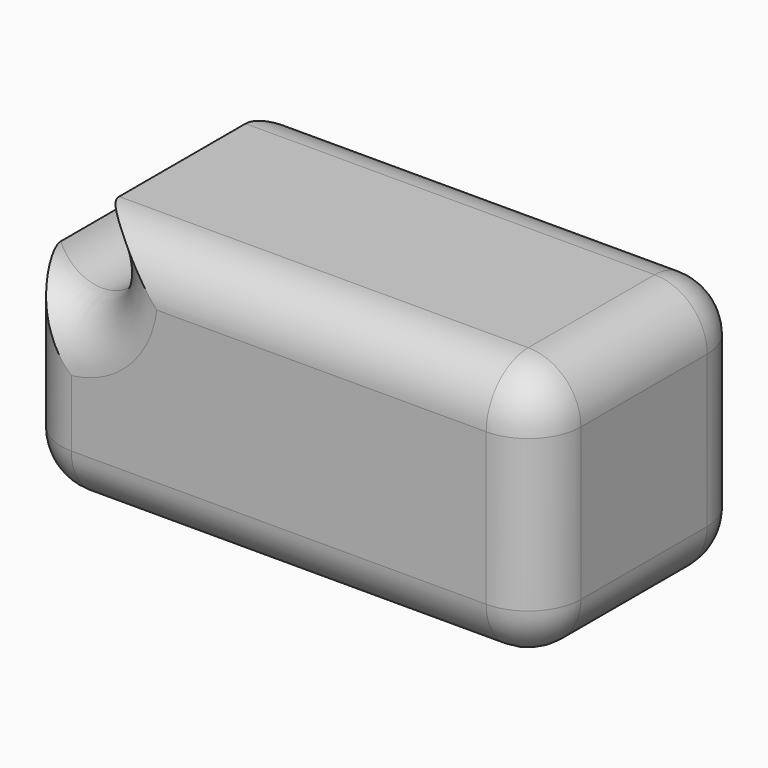
from build123d import *

# Parameters (mm, degrees)
F1_DEPTH     = 25.4
F2_T1_DEPTH  = 69.9704050186
F2_T3_DEPTH  = 26.8039856385
F2_T5_DEPTH  = 57.8223550216
F2_T7_DEPTH  = 50.2159356415
F2_T9_DEPTH  = 15.24
F2_S13_W     = 5.08
F2_S13_H     = 5.08
F2_T14_DEPTH = 5.08
F2_S19_W     = 5.08
F2_S19_H     = 5.08
F2_T20_DEPTH = 5.08
F2_T24_ANGLE = 359.64
F3_T1_DEPTH  = 15.24
F3_T3_DEPTH  = 52.1904050186
F3_S7_W      = 5.08
F3_S7_H      = 5.08
F3_T8_DEPTH  = 5.08
F3_T12_ANGLE = 89.9999999979
F4_T1_DEPTH  = 15.24
F4_S5_W      = 5.08
F4_S5_H      = 5.08
F4_T6_DEPTH  = 5.08
F4_S11_W     = 5.08
F4_S11_H     = 5.08
F4_T12_DEPTH = 5.08


# Not quite as in the source:
# - a fillet or chamfer that OpenCascade refuses, or shapes differently, is made with other operations: its cross-section is extruded or revolved along the edge and cut away or added


with BuildPart() as f1:
    # F0 (on Front) → F1 (new body)
    with BuildSketch(Plane.XZ):
        with BuildLine():
            Line((3.1376483385, 38.9353483915), (-41.4327566801, 38.9353483915))
            ThreePointArc((-41.4327566801, 38.9353483915), (-39.4863101259, 37.3460437845), (-38.7548631728, 34.9419787526))
            ThreePointArc((-38.7548631728, 34.9419787526), (-42.236270886, 30.7070512215), (-47.0647066832, 33.3033983885))
            Line((-47.0647066832, 33.3033983885), (-47.0647066832, 14.11941275))
            Line((-47.0647066832, 14.11941275), (3.1376483385, 14.11941275))
            Line((3.1376483385, 14.11941275), (3.1376483385, 38.9353483915))
        make_face()
    extrude(amount=F1_DEPTH)

    # F2: fillet of radius 5.08 on 9 edges, made by hand

    # F2_s2 → F2_t1 (cut)
    with BuildSketch(Plane.YZ.offset(-54.1327566801)):
        with BuildLine():
            ThreePointArc((-20.32, 38.9353483915), (-23.9121024484, 37.44745084), (-25.4, 33.8553483915))
            Line((-25.4, 33.8553483915), (-25.4, 38.9353483915))
            Line((-25.4, 38.9353483915), (-20.32, 38.9353483915))
        make_face()
    extrude(amount=F2_T1_DEPTH, mode=Mode.SUBTRACT)

    # F2_s4 → F2_t3 (cut)
    with BuildSketch(Plane.XY.offset(19.19941275)):
        with BuildLine():
            ThreePointArc((-41.9847066832, -25.4), (-45.5768091316, -23.9121024484), (-47.0647066832, -20.32))
            Line((-47.0647066832, -20.32), (-47.0647066832, -25.4))
            Line((-47.0647066832, -25.4), (-41.9847066832, -25.4))
        make_face()
        with BuildLine():
            ThreePointArc((-47.0647066832, -5.08), (-45.5768091316, -1.4878975516), (-41.9847066832, 0))
            Line((-41.9847066832, 0), (-47.0647066832, 0))
            Line((-47.0647066832, 0), (-47.0647066832, -5.08))
        make_face()
    extrude(amount=F2_T3_DEPTH, mode=Mode.SUBTRACT)

    # F2_s6 → F2_t5 (cut)
    with BuildSketch(Plane.YZ.offset(-41.9847066832)):
        with BuildLine():
            ThreePointArc((-25.4, 19.19941275), (-23.9121024484, 15.6073103016), (-20.32, 14.11941275))
            Line((-20.32, 14.11941275), (-25.4, 14.11941275))
            Line((-25.4, 14.11941275), (-25.4, 19.19941275))
        make_face()
        with BuildLine():
            ThreePointArc((-5.08, 14.11941275), (-1.4878975516, 15.6073103016), (0, 19.19941275))
            Line((0, 19.19941275), (0, 14.11941275))
            Line((0, 14.11941275), (-5.08, 14.11941275))
        make_face()
    extrude(amount=F2_T5_DEPTH, mode=Mode.SUBTRACT)

    # F2_s8 → F2_t7 (cut)
    with BuildSketch(Plane.XY.offset(1.41941275)):
        with BuildLine():
            ThreePointArc((-1.9423516615, -25.4), (1.6497507869, -23.9121024484), (3.1376483385, -20.32))
            Line((3.1376483385, -20.32), (3.1376483385, -25.4))
            Line((3.1376483385, -25.4), (-1.9423516615, -25.4))
        make_face()
        with BuildLine():
            ThreePointArc((-1.9423516615, 0), (1.6497507869, -1.4878975516), (3.1376483385, -5.08))
            Line((3.1376483385, -5.08), (3.1376483385, 0))
            Line((3.1376483385, 0), (-1.9423516615, 0))
        make_face()
    extrude(amount=F2_T7_DEPTH, mode=Mode.SUBTRACT)

    # F2_s10 → F2_t9 (cut)
    with BuildSketch(Plane.XZ.offset(5.08)):
        with BuildLine():
            ThreePointArc((-41.9847066832, 14.11941275), (-45.5768091316, 15.6073103016), (-47.0647066832, 19.19941275))
            Line((-47.0647066832, 19.19941275), (-47.0647066832, 14.11941275))
            Line((-47.0647066832, 14.11941275), (-41.9847066832, 14.11941275))
        make_face()
    extrude(amount=F2_T9_DEPTH, mode=Mode.SUBTRACT)


with BuildPart() as f2_tool12:
    # F2_s13 → F2_t14 (new body)
    with BuildSketch(Plane.XZ.offset(20.32)):
        with Locations((-44.5247066832, 16.65941275)):
            Rectangle(F2_S13_W, F2_S13_H)
    extrude(amount=F2_T14_DEPTH)

    # F2_s15 → F2_t16 (revolve, cut)
    with BuildSketch(Plane(origin=(-41.9847066832, -20.32, 19.19941275), x_dir=(0.7071067812, 0, 0.7071067812), z_dir=(0.7071067812, 0, -0.7071067812))):
        with BuildLine():
            ThreePointArc((0, -5.08), (5.08, 0), (0, 5.08))
            Line((0, 5.08), (0, -5.08))
        make_face()
    revolve(axis=Axis((-41.9847066832, -20.32, 19.19941275), (0, -1, 0)), mode=Mode.SUBTRACT)


with BuildPart() as f1_1:
    add(f1.part)

    # F2_t11: cut F2_tool12
    add(f2_tool12.part, mode=Mode.SUBTRACT)


with BuildPart() as f2_tool18:
    # F2_s19 → F2_t20 (new body)
    with BuildSketch(Plane.XY.offset(19.19941275)):
        with Locations((-44.5247066832, -2.54)):
            Rectangle(F2_S19_W, F2_S19_H)
    extrude(amount=-F2_T20_DEPTH)

    # F2_s21 → F2_t22 (revolve, cut)
    with BuildSketch(Plane(origin=(-41.9847066832, -5.08, 19.19941275), x_dir=(0.7071067812, -0.7071067812, 0), z_dir=(0.7071067812, 0.7071067812, 0))):
        with BuildLine():
            ThreePointArc((0, -5.08), (5.08, 0), (0, 5.08))
            Line((0, 5.08), (0, -5.08))
        make_face()
    revolve(axis=Axis((-41.9847066832, -5.08, 19.19941275), (0, 0, -1)), mode=Mode.SUBTRACT)


with BuildPart() as f1_2:
    add(f1_1.part)

    # F2_t17: cut F2_tool18
    add(f2_tool18.part, mode=Mode.SUBTRACT)

    # F2_s23 → F2_t24 (revolve, cut)
    with BuildSketch(Plane(origin=(-3.9297123025, 0, -3.9544813087), x_dir=(0, 1, 0), z_dir=(0.7048818539, 0, 0.7093247296))):
        with BuildLine():
            ThreePointArc((-25.4, 64.5780051362), (-23.9121024484, 60.9859026878), (-20.32, 59.4980051362))
            Line((-20.32, 59.4980051362), (-25.4, 59.4980051362))
            Line((-25.4, 59.4980051362), (-25.4, 64.5780051362))
        make_face()
    revolve(axis=Axis((-43.0713370442, -25.4, 34.9419787526), (0, -1, 0)), revolution_arc=F2_T24_ANGLE, mode=Mode.SUBTRACT)

    # F3: fillet of radius 5.08 on 1 edges, made by hand

    # F3_s2 → F3_t1 (cut)
    with BuildSketch(Plane.XZ.offset(5.08)):
        with BuildLine():
            ThreePointArc((-1.9423516615, 38.9353483915), (1.6497507869, 37.44745084), (3.1376483385, 33.8553483915))
            Line((3.1376483385, 33.8553483915), (3.1376483385, 38.9353483915))
            Line((3.1376483385, 38.9353483915), (-1.9423516615, 38.9353483915))
        make_face()
    extrude(amount=F3_T1_DEPTH, mode=Mode.SUBTRACT)

    # F3_s4 → F3_t3 (cut)
    with BuildSketch(Plane.YZ.offset(-54.1327566801)):
        with BuildLine():
            ThreePointArc((-5.08, 38.9353483915), (-1.4878975516, 37.44745084), (0, 33.8553483915))
            Line((0, 33.8553483915), (0, 38.9353483915))
            Line((0, 38.9353483915), (-5.08, 38.9353483915))
        make_face()
    extrude(amount=F3_T3_DEPTH, mode=Mode.SUBTRACT)


with BuildPart() as f3_tool6:
    # F3_s7 → F3_t8 (new body)
    with BuildSketch(Plane.XY.offset(33.8553483915)):
        with Locations((0.5976483385, -22.86)):
            Rectangle(F3_S7_W, F3_S7_H)
    extrude(amount=F3_T8_DEPTH)

    # F3_s9 → F3_t10 (revolve, cut)
    with BuildSketch(Plane(origin=(-1.9423516615, -20.32, 33.8553483915), x_dir=(-0.7071067812, 0.7071067812, 0), z_dir=(0.7071067812, 0.7071067812, 0))):
        with BuildLine():
            ThreePointArc((0, -5.08), (5.08, 0), (0, 5.08))
            Line((0, 5.08), (0, -5.08))
        make_face()
    revolve(axis=Axis((-1.9423516615, -20.32, 33.8553483915), (0, 0, 1)), mode=Mode.SUBTRACT)


with BuildPart() as f1_3:
    add(f1_2.part)

    # F3_t5: cut F3_tool6
    add(f3_tool6.part, mode=Mode.SUBTRACT)

    # F3_s11 → F3_t12 (revolve, cut)
    with BuildSketch(Plane.YZ.offset(-1.9423516616)):
        with BuildLine():
            ThreePointArc((-5.08, 38.9353483915), (-1.4878975516, 37.44745084), (0, 33.8553483915))
            Line((0, 33.8553483915), (0, 38.9353483915))
            Line((0, 38.9353483915), (-5.08, 38.9353483915))
        make_face()
    revolve(axis=Axis((-1.9423516616, -5.0800000001, 38.9353483915), (0, 0, -1)), revolution_arc=F3_T12_ANGLE, mode=Mode.SUBTRACT)

    # F4: fillet of radius 5.08 on 1 edges, made by hand

    # F4_s2 → F4_t1 (cut)
    with BuildSketch(Plane.XZ.offset(5.08)):
        with BuildLine():
            ThreePointArc((3.1376483385, 19.19941275), (1.6497507869, 15.6073103016), (-1.9423516615, 14.11941275))
            Line((-1.9423516615, 14.11941275), (3.1376483385, 14.11941275))
            Line((3.1376483385, 14.11941275), (3.1376483385, 19.19941275))
        make_face()
    extrude(amount=F4_T1_DEPTH, mode=Mode.SUBTRACT)


with BuildPart() as f4_tool4:
    # F4_s5 → F4_t6 (new body)
    with BuildSketch(Plane.YZ.offset(-1.9423516615)):
        with Locations((-2.54, 16.65941275)):
            Rectangle(F4_S5_W, F4_S5_H)
    extrude(amount=F4_T6_DEPTH)

    # F4_s7 → F4_t8 (revolve, cut)
    with BuildSketch(Plane(origin=(-1.9423516615, -5.08, 19.19941275), x_dir=(0, -0.7071067812, 0.7071067812), z_dir=(0, 0.7071067812, 0.7071067812))):
        with BuildLine():
            ThreePointArc((0, -5.08), (5.08, 0), (0, 5.08))
            Line((0, 5.08), (0, -5.08))
        make_face()
    revolve(axis=Axis((-1.9423516615, -5.08, 19.19941275), (1, 0, 0)), mode=Mode.SUBTRACT)


with BuildPart() as f1_4:
    add(f1_3.part)

    # F4_t3: cut F4_tool4
    add(f4_tool4.part, mode=Mode.SUBTRACT)


with BuildPart() as f4_tool10:
    # F4_s11 → F4_t12 (new body)
    with BuildSketch(Plane.YZ.offset(-1.9423516615)):
        with Locations((-22.86, 16.65941275)):
            Rectangle(F4_S11_W, F4_S11_H)
    extrude(amount=F4_T12_DEPTH)

    # F4_s13 → F4_t14 (revolve, cut)
    with BuildSketch(Plane(origin=(-1.9423516615, -20.32, 19.19941275), x_dir=(0, 0.7071067812, 0.7071067812), z_dir=(0, 0.7071067812, -0.7071067812))):
        with BuildLine():
            ThreePointArc((0, -5.08), (5.08, 0), (0, 5.08))
            Line((0, 5.08), (0, -5.08))
        make_face()
    revolve(axis=Axis((-1.9423516615, -20.32, 19.19941275), (1, 0, 0)), mode=Mode.SUBTRACT)


with BuildPart() as f1_5:
    add(f1_4.part)

    # F4_t9: cut F4_tool10
    add(f4_tool10.part, mode=Mode.SUBTRACT)


solid = f1_5.part
